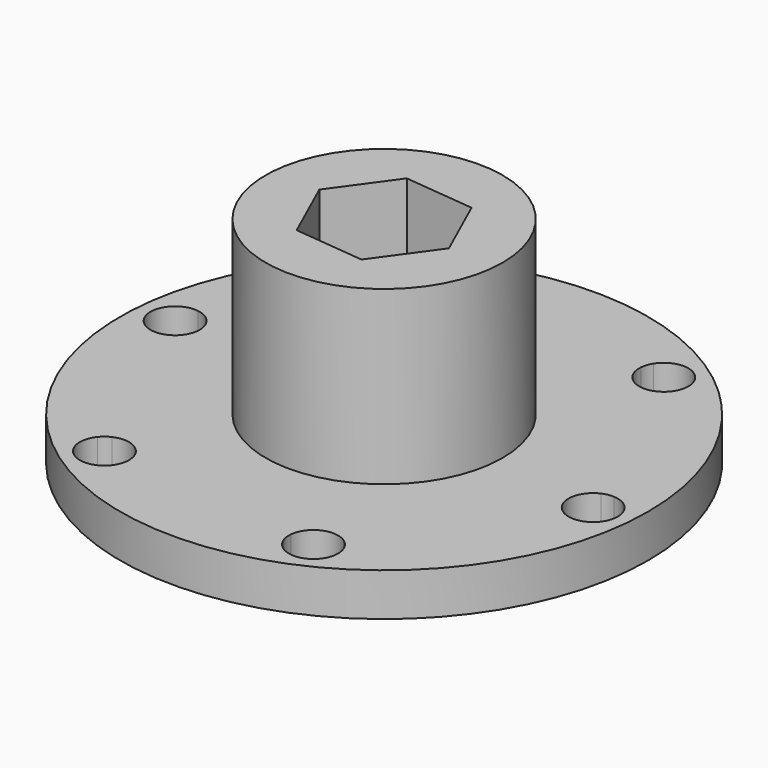
from build123d import *

# Parameters (mm, degrees)
F0_R     = 27.305
F0_R_2   = 14.2875
F0_R_3   = 9.271
F1_DEPTH = 4.445
F2_R     = 12.2555
F3_DEPTH = 17.78
F4_DEPTH = 2.54
F5_DEPTH = 1.27
F7_DEPTH = 25.4
F8_DEPTH = 25.4


# Not quite as in the source:
# - a feature names something its author has since deleted; it is built from what else it names


with BuildPart() as f1:
    # F0 (on Top) → F1 (new body)
    with BuildSketch(Plane.XY):
        Circle(F0_R)
        with BuildLine():
            ThreePointArc((25.93093901, -2.2088452252), (25.0490643413, -4.1329607067), (23.015804848, -4.7209905953))
            ThreePointArc((23.015804848, -4.7209905953), (19.1527247884, -13.6083855831), (12.0313699631, -20.180712619))
            ThreePointArc((12.0313699631, -20.180712619), (12.2486833913, -20.753455716), (12.3225534269, -21.3615700137))
            ThreePointArc((12.3225534269, -21.3615700137), (10.2564743458, -23.856965566), (7.4194046374, -22.2927669845))
            ThreePointArc((7.4194046374, -22.2927669845), (-2.2088452252, -23.39093901), (-11.461324813, -20.5098283399))
            ThreePointArc((-11.461324813, -20.5098283399), (-15.0795624029, -21.2232896304), (-15.5964002105, -17.5717763892))
            ThreePointArc((-15.5964002105, -17.5717763892), (-21.3615700137, -9.7825534269), (-23.4926947761, -0.3291157209))
            ThreePointArc((-23.4926947761, -0.3291157209), (-25.9196891733, 2.4476393036), (-23.015804848, 4.7209905953))
            ThreePointArc((-23.015804848, 4.7209905953), (-19.1527247884, 13.6083855831), (-12.0313699631, 20.180712619))
            ThreePointArc((-12.0313699631, 20.180712619), (-10.8401267704, 23.6709289341), (-7.4194046374, 22.2927669845))
            ThreePointArc((-7.4194046374, 22.2927669845), (2.2088452252, 23.39093901), (11.461324813, 20.5098283399))
            ThreePointArc((11.461324813, 20.5098283399), (14.3148081351, 21.5925131354), (16.1483855831, 19.1527247884))
            ThreePointArc((16.1483855831, 19.1527247884), (16.0064219833, 18.3154545673), (15.5964002105, 17.5717763892))
            ThreePointArc((15.5964002105, 17.5717763892), (21.3615700137, 9.7825534269), (23.4926947761, 0.3291157209))
            ThreePointArc((23.4926947761, 0.3291157209), (25.2226130593, -0.4491378129), (25.93093901, -2.2088452252))
        make_face(mode=Mode.SUBTRACT)
        with BuildLine():
            ThreePointArc((21.9197621902, -4.2794100672), (20.8621888468, -1.9700511468), (22.3333656666, 0.1005136952))
            Line((22.3333656666, 0.1005136952), (14.6659589265, 16.843365868))
            ThreePointArc((14.6659589265, 16.843365868), (12.1372087633, 17.0821599464), (11.0796354198, 19.3915188668))
            Line((11.0796354198, 19.3915188668), (-7.2538032637, 21.1227759353))
            ThreePointArc((-7.2538032637, 21.1227759353), (-8.7249800835, 19.0522110933), (-11.2537302467, 19.2910051717))
            Line((-11.2537302467, 19.2910051717), (-21.9197621902, 4.2794100672))
            ThreePointArc((-21.9197621902, 4.2794100672), (-21.1339067637, 3.3739226642), (-20.85093901, 2.2088452252))
            ThreePointArc((-20.85093901, 2.2088452252), (-21.2534362273, 0.8367366822), (-22.3333656666, -0.1005136952))
            Line((-22.3333656666, -0.1005136952), (-14.6659589265, -16.843365868))
            ThreePointArc((-14.6659589265, -16.843365868), (-12.2362770401, -17.0152220057), (-11.0683855831, -19.1527247884))
            ThreePointArc((-11.0683855831, -19.1527247884), (-11.0711996011, -19.2722542521), (-11.0796354198, -19.3915188668))
            Line((-11.0796354198, -19.3915188668), (7.2538032637, -21.1227759353))
            ThreePointArc((7.2538032637, -21.1227759353), (8.7249800835, -19.0522110933), (11.2537302467, -19.2910051717))
            Line((11.2537302467, -19.2910051717), (21.9197621902, -4.2794100672))
        make_face()
        Circle(F0_R_2, mode=Mode.SUBTRACT)
        Circle(F0_R_2)
        Circle(F0_R_3, mode=Mode.SUBTRACT)
        Circle(F0_R_3)
        with BuildLine():
            Line((14.6659589265, 16.843365868), (22.3333656666, 0.1005136952))
            ThreePointArc((22.3333656666, 0.1005136952), (22.8995516558, 0.2831697162), (23.4926947761, 0.3291157209))
            ThreePointArc((23.4926947761, 0.3291157209), (21.3615700137, 9.7825534269), (15.5964002105, 17.5717763892))
            ThreePointArc((15.5964002105, 17.5717763892), (15.1741272585, 17.152711537), (14.6659589265, 16.843365868))
        make_face()
        with BuildLine():
            Line((-7.2538032637, 21.1227759353), (11.0796354198, 19.3915188668))
            ThreePointArc((11.0796354198, 19.3915188668), (11.2045436601, 19.9731783273), (11.461324813, 20.5098283399))
            ThreePointArc((11.461324813, 20.5098283399), (2.2088452252, 23.39093901), (-7.4194046374, 22.2927669845))
            ThreePointArc((-7.4194046374, 22.2927669845), (-7.2871578746, 21.8354909325), (-7.2425534269, 21.3615700137))
            ThreePointArc((-7.2425534269, 21.3615700137), (-7.2453674449, 21.24204055), (-7.2538032637, 21.1227759353))
        make_face()
        with BuildLine():
            Line((-21.9197621902, 4.2794100672), (-11.2537302467, 19.2910051717))
            ThreePointArc((-11.2537302467, 19.2910051717), (-11.6950079957, 19.6900086111), (-12.0313699631, 20.180712619))
            ThreePointArc((-12.0313699631, 20.180712619), (-19.1527247884, 13.6083855831), (-23.015804848, 4.7209905953))
            ThreePointArc((-23.015804848, 4.7209905953), (-22.441747564, 4.5648239176), (-21.9197621902, 4.2794100672))
        make_face()
        with BuildLine():
            ThreePointArc((-23.4926947761, -0.3291157209), (-21.3615700137, -9.7825534269), (-15.5964002105, -17.5717763892))
            ThreePointArc((-15.5964002105, -17.5717763892), (-15.1741272585, -17.152711537), (-14.6659589265, -16.843365868))
            Line((-14.6659589265, -16.843365868), (-22.3333656666, -0.1005136952))
            ThreePointArc((-22.3333656666, -0.1005136952), (-22.8995516558, -0.2831697162), (-23.4926947761, -0.3291157209))
        make_face()
        with BuildLine():
            ThreePointArc((7.4194046374, -22.2927669845), (7.2676203056, -21.7175354546), (7.2538032637, -21.1227759353))
            Line((7.2538032637, -21.1227759353), (-11.0796354198, -19.3915188668))
            ThreePointArc((-11.0796354198, -19.3915188668), (-11.2045436601, -19.9731783273), (-11.461324813, -20.5098283399))
            ThreePointArc((-11.461324813, -20.5098283399), (-2.2088452252, -23.39093901), (7.4194046374, -22.2927669845))
        make_face()
        with BuildLine():
            ThreePointArc((12.0313699631, -20.180712619), (19.1527247884, -13.6083855831), (23.015804848, -4.7209905953))
            ThreePointArc((23.015804848, -4.7209905953), (22.441747564, -4.5648239176), (21.9197621902, -4.2794100672))
            Line((21.9197621902, -4.2794100672), (11.2537302467, -19.2910051717))
            ThreePointArc((11.2537302467, -19.2910051717), (11.6950079957, -19.6900086111), (12.0313699631, -20.180712619))
        make_face()
        with BuildLine():
            ThreePointArc((-11.2537302467, 19.2910051717), (-8.7249800835, 19.0522110933), (-7.2538032637, 21.1227759353))
            Line((-7.2538032637, 21.1227759353), (-9.7825534269, 21.3615700137))
            Line((-9.7825534269, 21.3615700137), (-11.2537302467, 19.2910051717))
        make_face()
        with BuildLine():
            ThreePointArc((-20.85093901, 2.2088452252), (-21.1339067637, 3.3739226642), (-21.9197621902, 4.2794100672))
            Line((-21.9197621902, 4.2794100672), (-23.39093901, 2.2088452252))
            Line((-23.39093901, 2.2088452252), (-22.3333656666, -0.1005136952))
            ThreePointArc((-22.3333656666, -0.1005136952), (-21.2534362273, 0.8367366822), (-20.85093901, 2.2088452252))
        make_face()
        with BuildLine():
            Line((-13.6083855831, -19.1527247884), (-11.0796354198, -19.3915188668))
            ThreePointArc((-11.0796354198, -19.3915188668), (-11.0711996011, -19.2722542521), (-11.0683855831, -19.1527247884))
            ThreePointArc((-11.0683855831, -19.1527247884), (-12.2362770401, -17.0152220057), (-14.6659589265, -16.843365868))
            Line((-14.6659589265, -16.843365868), (-13.6083855831, -19.1527247884))
        make_face()
        with BuildLine():
            Line((9.7825534269, -21.3615700137), (11.2537302467, -19.2910051717))
            ThreePointArc((11.2537302467, -19.2910051717), (8.7249800835, -19.0522110933), (7.2538032637, -21.1227759353))
            Line((7.2538032637, -21.1227759353), (9.7825534269, -21.3615700137))
        make_face()
        with BuildLine():
            Line((21.9197621902, -4.2794100672), (23.39093901, -2.2088452252))
            Line((23.39093901, -2.2088452252), (22.3333656666, 0.1005136952))
            ThreePointArc((22.3333656666, 0.1005136952), (20.8621888468, -1.9700511468), (21.9197621902, -4.2794100672))
        make_face()
        with BuildLine():
            ThreePointArc((11.0796354198, 19.3915188668), (12.1372087633, 17.0821599464), (14.6659589265, 16.843365868))
            Line((14.6659589265, 16.843365868), (13.6083855831, 19.1527247884))
            Line((13.6083855831, 19.1527247884), (11.0796354198, 19.3915188668))
        make_face()
        with BuildLine():
            Line((13.6083855831, 19.1527247884), (14.6659589265, 16.843365868))
            ThreePointArc((14.6659589265, 16.843365868), (15.1741272585, 17.152711537), (15.5964002105, 17.5717763892))
            ThreePointArc((15.5964002105, 17.5717763892), (14.6237726929, 18.3891353039), (13.6083855831, 19.1527247884))
        make_face()
        with BuildLine():
            Line((11.0796354198, 19.3915188668), (13.6083855831, 19.1527247884))
            ThreePointArc((13.6083855831, 19.1527247884), (12.5532078509, 19.8603121237), (11.461324813, 20.5098283399))
            ThreePointArc((11.461324813, 20.5098283399), (11.2045436601, 19.9731783273), (11.0796354198, 19.3915188668))
        make_face()
        with BuildLine():
            Line((-9.7825534269, 21.3615700137), (-7.2538032637, 21.1227759353))
            ThreePointArc((-7.2538032637, 21.1227759353), (-7.2453674449, 21.24204055), (-7.2425534269, 21.3615700137))
            ThreePointArc((-7.2425534269, 21.3615700137), (-7.2871578746, 21.8354909325), (-7.4194046374, 22.2927669845))
            ThreePointArc((-7.4194046374, 22.2927669845), (-8.6135719804, 21.8591263032), (-9.7825534269, 21.3615700137))
        make_face()
        with BuildLine():
            Line((-11.2537302467, 19.2910051717), (-9.7825534269, 21.3615700137))
            ThreePointArc((-9.7825534269, 21.3615700137), (-10.9229309008, 20.8015529597), (-12.0313699631, 20.180712619))
            ThreePointArc((-12.0313699631, 20.180712619), (-11.6950079957, 19.6900086111), (-11.2537302467, 19.2910051717))
        make_face()
        with BuildLine():
            Line((-23.39093901, 2.2088452252), (-21.9197621902, 4.2794100672))
            ThreePointArc((-21.9197621902, 4.2794100672), (-22.441747564, 4.5648239176), (-23.015804848, 4.7209905953))
            ThreePointArc((-23.015804848, 4.7209905953), (-23.2373446733, 3.4699909992), (-23.39093901, 2.2088452252))
        make_face()
        with BuildLine():
            ThreePointArc((-23.39093901, 2.2088452252), (-23.4761387517, 0.941240836), (-23.4926947761, -0.3291157209))
            ThreePointArc((-23.4926947761, -0.3291157209), (-22.8995516558, -0.2831697162), (-22.3333656666, -0.1005136952))
            Line((-22.3333656666, -0.1005136952), (-23.39093901, 2.2088452252))
        make_face()
        with BuildLine():
            ThreePointArc((-15.5964002105, -17.5717763892), (-14.6237726929, -18.3891353039), (-13.6083855831, -19.1527247884))
            Line((-13.6083855831, -19.1527247884), (-14.6659589265, -16.843365868))
            ThreePointArc((-14.6659589265, -16.843365868), (-15.1741272585, -17.152711537), (-15.5964002105, -17.5717763892))
        make_face()
        with BuildLine():
            ThreePointArc((-11.461324813, -20.5098283399), (-11.2045436601, -19.9731783273), (-11.0796354198, -19.3915188668))
            Line((-11.0796354198, -19.3915188668), (-13.6083855831, -19.1527247884))
            ThreePointArc((-13.6083855831, -19.1527247884), (-12.5532078509, -19.8603121237), (-11.461324813, -20.5098283399))
        make_face()
        with BuildLine():
            ThreePointArc((7.4194046374, -22.2927669845), (8.6135719804, -21.8591263032), (9.7825534269, -21.3615700137))
            Line((9.7825534269, -21.3615700137), (7.2538032637, -21.1227759353))
            ThreePointArc((7.2538032637, -21.1227759353), (7.2676203056, -21.7175354546), (7.4194046374, -22.2927669845))
        make_face()
        with BuildLine():
            ThreePointArc((9.7825534269, -21.3615700137), (10.9229309008, -20.8015529597), (12.0313699631, -20.180712619))
            ThreePointArc((12.0313699631, -20.180712619), (11.6950079957, -19.6900086111), (11.2537302467, -19.2910051717))
            Line((11.2537302467, -19.2910051717), (9.7825534269, -21.3615700137))
        make_face()
        with BuildLine():
            ThreePointArc((23.015804848, -4.7209905953), (23.2373446733, -3.4699909992), (23.39093901, -2.2088452252))
            Line((23.39093901, -2.2088452252), (21.9197621902, -4.2794100672))
            ThreePointArc((21.9197621902, -4.2794100672), (22.441747564, -4.5648239176), (23.015804848, -4.7209905953))
        make_face()
        with BuildLine():
            Line((22.3333656666, 0.1005136952), (23.39093901, -2.2088452252))
            ThreePointArc((23.39093901, -2.2088452252), (23.4689703336, -1.1056475386), (23.495, 0))
            ThreePointArc((23.495, 0), (23.494423687, 0.164561897), (23.4926947761, 0.3291157209))
            ThreePointArc((23.4926947761, 0.3291157209), (22.8995516558, 0.2831697162), (22.3333656666, 0.1005136952))
        make_face()
    extrude(amount=F1_DEPTH)

    # F2 (on face) → F3 (join)
    with BuildSketch(Plane.XY.offset(4.445)):
        Circle(F2_R)
    extrude(amount=F3_DEPTH)

    # F0 (on Top) → F4 (join)
    with BuildSketch(Plane.XY):
        Circle(F0_R_3)
    extrude(amount=-F4_DEPTH)

    # F0 (on Top) → F5 (join)
    with BuildSketch(Plane.XY):
        Circle(F0_R_2)
        Circle(F0_R_3, mode=Mode.SUBTRACT)
    extrude(amount=-F5_DEPTH)

    # F6 (on face) → F7 (cut)
    with BuildSketch(Plane.XY.offset(22.225)):
        Polygon((-4.2897580502, -5.9465375811), (3.0049735847, -6.6883082382), (7.2947316349, -0.741770657), (4.2897580502, 5.9465375811), (-3.0049735847, 6.6883082382), (-7.2947316349, 0.741770657), align=None)
    extrude(amount=-F7_DEPTH, mode=Mode.SUBTRACT)

    # F0 (on Top) → F8 (cut)
    with BuildSketch(Plane.XY):
        with BuildLine():
            ThreePointArc((11.0796354198, 19.3915188668), (12.1372087633, 17.0821599464), (14.6659589265, 16.843365868))
            Line((14.6659589265, 16.843365868), (13.6083855831, 19.1527247884))
            Line((13.6083855831, 19.1527247884), (11.0796354198, 19.3915188668))
        make_face()
        with BuildLine():
            Line((13.6083855831, 19.1527247884), (14.6659589265, 16.843365868))
            ThreePointArc((14.6659589265, 16.843365868), (15.1741272585, 17.152711537), (15.5964002105, 17.5717763892))
            ThreePointArc((15.5964002105, 17.5717763892), (14.6237726929, 18.3891353039), (13.6083855831, 19.1527247884))
        make_face()
        with BuildLine():
            Line((11.0796354198, 19.3915188668), (13.6083855831, 19.1527247884))
            ThreePointArc((13.6083855831, 19.1527247884), (12.5532078509, 19.8603121237), (11.461324813, 20.5098283399))
            ThreePointArc((11.461324813, 20.5098283399), (11.2045436601, 19.9731783273), (11.0796354198, 19.3915188668))
        make_face()
        with BuildLine():
            Line((-23.39093901, 2.2088452252), (-21.9197621902, 4.2794100672))
            ThreePointArc((-21.9197621902, 4.2794100672), (-22.441747564, 4.5648239176), (-23.015804848, 4.7209905953))
            ThreePointArc((-23.015804848, 4.7209905953), (-23.2373446733, 3.4699909992), (-23.39093901, 2.2088452252))
        make_face()
        with BuildLine():
            ThreePointArc((-20.85093901, 2.2088452252), (-21.1339067637, 3.3739226642), (-21.9197621902, 4.2794100672))
            Line((-21.9197621902, 4.2794100672), (-23.39093901, 2.2088452252))
            Line((-23.39093901, 2.2088452252), (-22.3333656666, -0.1005136952))
            ThreePointArc((-22.3333656666, -0.1005136952), (-21.2534362273, 0.8367366822), (-20.85093901, 2.2088452252))
        make_face()
        with BuildLine():
            ThreePointArc((-23.39093901, 2.2088452252), (-23.4761387517, 0.941240836), (-23.4926947761, -0.3291157209))
            ThreePointArc((-23.4926947761, -0.3291157209), (-22.8995516558, -0.2831697162), (-22.3333656666, -0.1005136952))
            Line((-22.3333656666, -0.1005136952), (-23.39093901, 2.2088452252))
        make_face()
        with BuildLine():
            Line((-11.2537302467, 19.2910051717), (-9.7825534269, 21.3615700137))
            ThreePointArc((-9.7825534269, 21.3615700137), (-10.9229309008, 20.8015529597), (-12.0313699631, 20.180712619))
            ThreePointArc((-12.0313699631, 20.180712619), (-11.6950079957, 19.6900086111), (-11.2537302467, 19.2910051717))
        make_face()
        with BuildLine():
            ThreePointArc((-11.2537302467, 19.2910051717), (-8.7249800835, 19.0522110933), (-7.2538032637, 21.1227759353))
            Line((-7.2538032637, 21.1227759353), (-9.7825534269, 21.3615700137))
            Line((-9.7825534269, 21.3615700137), (-11.2537302467, 19.2910051717))
        make_face()
        with BuildLine():
            Line((-9.7825534269, 21.3615700137), (-7.2538032637, 21.1227759353))
            ThreePointArc((-7.2538032637, 21.1227759353), (-7.2453674449, 21.24204055), (-7.2425534269, 21.3615700137))
            ThreePointArc((-7.2425534269, 21.3615700137), (-7.2871578746, 21.8354909325), (-7.4194046374, 22.2927669845))
            ThreePointArc((-7.4194046374, 22.2927669845), (-8.6135719804, 21.8591263032), (-9.7825534269, 21.3615700137))
        make_face()
        with BuildLine():
            Line((-13.6083855831, -19.1527247884), (-11.0796354198, -19.3915188668))
            ThreePointArc((-11.0796354198, -19.3915188668), (-11.0711996011, -19.2722542521), (-11.0683855831, -19.1527247884))
            ThreePointArc((-11.0683855831, -19.1527247884), (-12.2362770401, -17.0152220057), (-14.6659589265, -16.843365868))
            Line((-14.6659589265, -16.843365868), (-13.6083855831, -19.1527247884))
        make_face()
        with BuildLine():
            ThreePointArc((-11.461324813, -20.5098283399), (-11.2045436601, -19.9731783273), (-11.0796354198, -19.3915188668))
            Line((-11.0796354198, -19.3915188668), (-13.6083855831, -19.1527247884))
            ThreePointArc((-13.6083855831, -19.1527247884), (-12.5532078509, -19.8603121237), (-11.461324813, -20.5098283399))
        make_face()
        with BuildLine():
            ThreePointArc((-15.5964002105, -17.5717763892), (-14.6237726929, -18.3891353039), (-13.6083855831, -19.1527247884))
            Line((-13.6083855831, -19.1527247884), (-14.6659589265, -16.843365868))
            ThreePointArc((-14.6659589265, -16.843365868), (-15.1741272585, -17.152711537), (-15.5964002105, -17.5717763892))
        make_face()
        with BuildLine():
            Line((9.7825534269, -21.3615700137), (11.2537302467, -19.2910051717))
            ThreePointArc((11.2537302467, -19.2910051717), (8.7249800835, -19.0522110933), (7.2538032637, -21.1227759353))
            Line((7.2538032637, -21.1227759353), (9.7825534269, -21.3615700137))
        make_face()
        with BuildLine():
            ThreePointArc((7.4194046374, -22.2927669845), (8.6135719804, -21.8591263032), (9.7825534269, -21.3615700137))
            Line((9.7825534269, -21.3615700137), (7.2538032637, -21.1227759353))
            ThreePointArc((7.2538032637, -21.1227759353), (7.2676203056, -21.7175354546), (7.4194046374, -22.2927669845))
        make_face()
        with BuildLine():
            ThreePointArc((9.7825534269, -21.3615700137), (10.9229309008, -20.8015529597), (12.0313699631, -20.180712619))
            ThreePointArc((12.0313699631, -20.180712619), (11.6950079957, -19.6900086111), (11.2537302467, -19.2910051717))
            Line((11.2537302467, -19.2910051717), (9.7825534269, -21.3615700137))
        make_face()
        with BuildLine():
            Line((21.9197621902, -4.2794100672), (23.39093901, -2.2088452252))
            Line((23.39093901, -2.2088452252), (22.3333656666, 0.1005136952))
            ThreePointArc((22.3333656666, 0.1005136952), (20.8621888468, -1.9700511468), (21.9197621902, -4.2794100672))
        make_face()
        with BuildLine():
            Line((22.3333656666, 0.1005136952), (23.39093901, -2.2088452252))
            ThreePointArc((23.39093901, -2.2088452252), (23.4689703336, -1.1056475386), (23.495, 0))
            ThreePointArc((23.495, 0), (23.494423687, 0.164561897), (23.4926947761, 0.3291157209))
            ThreePointArc((23.4926947761, 0.3291157209), (22.8995516558, 0.2831697162), (22.3333656666, 0.1005136952))
        make_face()
        with BuildLine():
            ThreePointArc((23.015804848, -4.7209905953), (23.2373446733, -3.4699909992), (23.39093901, -2.2088452252))
            Line((23.39093901, -2.2088452252), (21.9197621902, -4.2794100672))
            ThreePointArc((21.9197621902, -4.2794100672), (22.441747564, -4.5648239176), (23.015804848, -4.7209905953))
        make_face()
    extrude(amount=F8_DEPTH, mode=Mode.SUBTRACT)


solid = f1.part
